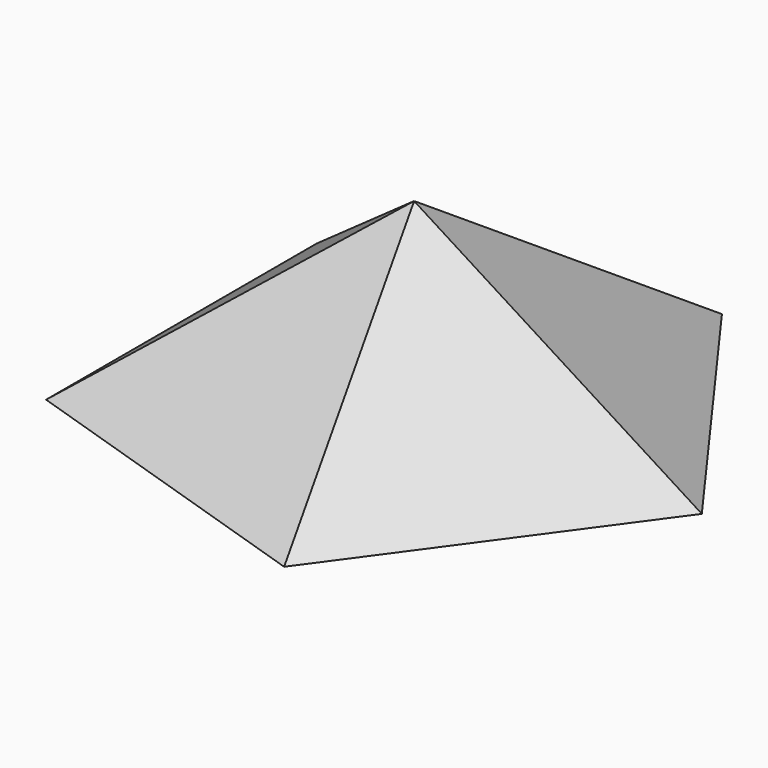
from build123d import *

# Parameters (mm, degrees)
F1_DEPTH = 27.178
F2_SIZE2 = 34.786244
F2_SIZE  = 27.17799


# Not quite as in the source:
# - a fillet or chamfer is up to 0.001 mm smaller than in the source, because OpenCascade refuses the exact size


with BuildPart() as f1:
    # F0 (on Top) → F1 (new body)
    with BuildSketch(Plane.XY):
        Polygon((-34.96010078, -25.4), (13.3535702478, -41.0980633142), (43.2130610643, 0), (13.3535702478, 41.0980633142), (-34.96010078, 25.4), align=None)
    extrude(amount=F1_DEPTH)

    # F2 (size 27.178 and 34.7862536797 in the source; OpenCascade refuses exactly that, so slightly less here)
    f2_edges = [f1.edges().sort_by_distance(p)[0] for p in [
        (28.283316, -20.549032, 27.178),
        (-10.803265, 33.249032, 27.178),
        (-34.960101, 0, 27.178),
        (-10.803265, -33.249032, 27.178),
        (28.283316, 20.549032, 27.178),
    ]]
    chamfer(f2_edges, length=F2_SIZE, length2=F2_SIZE2)


solid = f1.part
